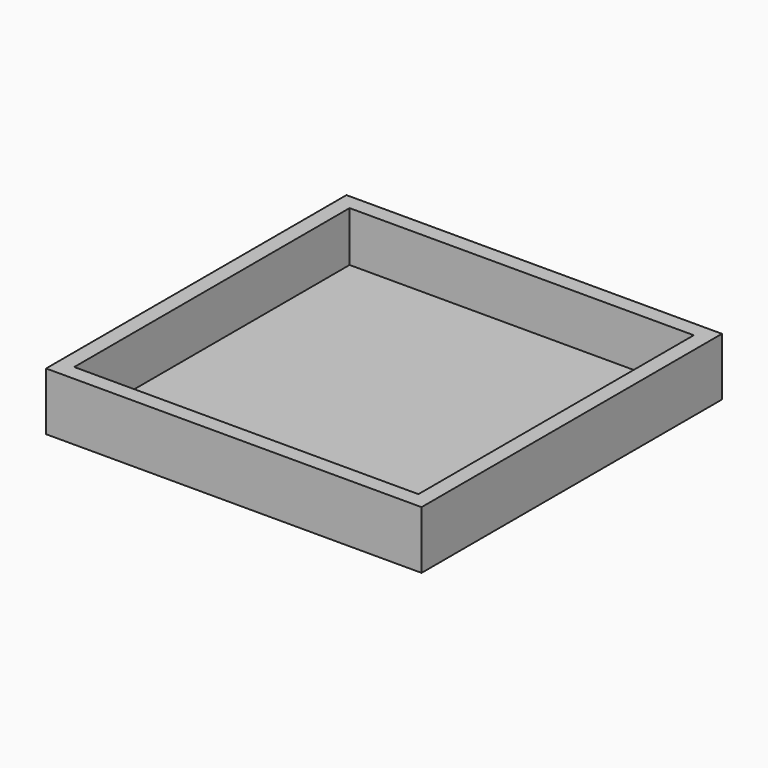
from build123d import *

# Parameters (mm, degrees)
F0_W     = 38.1
F0_H     = 38.1
F1_DEPTH = 0.79375
F2_W     = 38.1
F2_H     = 38.1
F2_W_2   = 34.925
F2_H_2   = 34.925
F3_DEPTH = 5.08


# Not quite as in the source:
# - the program builds the solid bodies; features that only make, move or delete a surface that nothing else refers to are left out


with BuildPart() as f1:
    # F0 (on Top) → F1 (new body)
    with BuildSketch(Plane.XY):
        with Locations((1.1546928436, 7.4534941071)):
            Rectangle(F0_W, F0_H)
    extrude(amount=F1_DEPTH)

    # F2 (on face) → F3 (join)
    with BuildSketch(Plane.XY.offset(0.79375)):
        with Locations((1.1546928436, 7.4534941071)):
            Rectangle(F2_W, F2_H)
        with Locations((1.1546928436, 7.4534941071)):
            Rectangle(F2_W_2, F2_H_2, mode=Mode.SUBTRACT)
    extrude(amount=F3_DEPTH)


solid = f1.part
